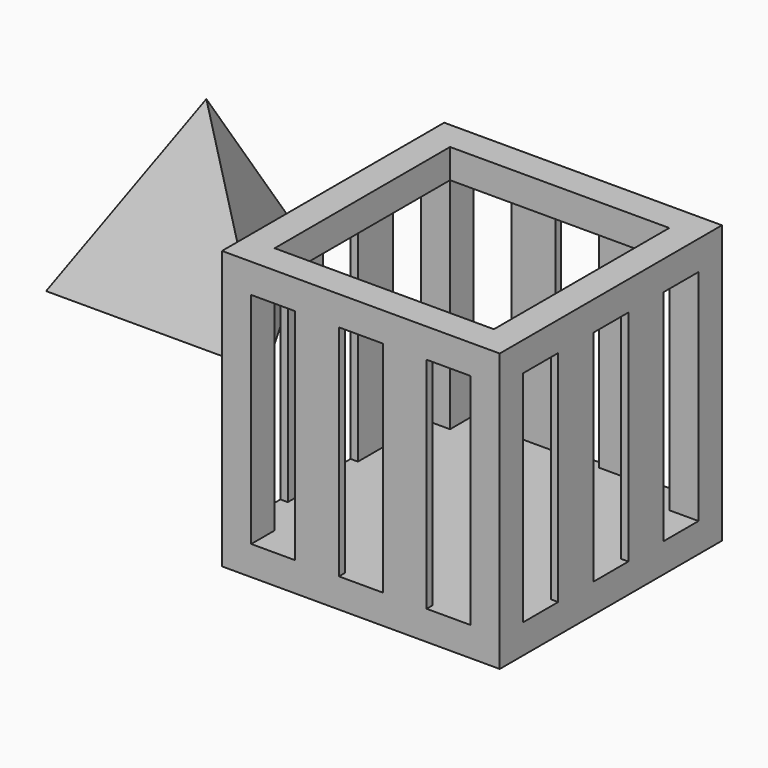
from build123d import *

# Parameters (mm, degrees)
F0_W      = 76
F0_H      = 76
F1_DEPTH  = 76
F2_W      = 60
F2_H      = 60
F3_DEPTH  = 68
F4_W      = 12
F4_H      = 60
F5_DEPTH  = 100
F6_W      = 12
F6_H      = 60
F7_DEPTH  = 6
F8_W      = 12
F8_H      = 60
F9_DEPTH  = 6
F10_W     = 12
F10_H     = 60
F11_DEPTH = 99
F12_W     = 12
F12_H     = 60
F13_DEPTH = 6
F14_W     = 12
F14_H     = 60
F15_DEPTH = 6
F17_DEPTH = 48.9897948557
F20_W     = 96.6173894703
F20_H     = 69.0555498004
F21_DEPTH = 25
F23_W     = 74.8236617073
F23_H     = 72.9810190387
F24_DEPTH = 25
F26_W     = 108.0368701369
F26_H     = 112.1664643288
F27_DEPTH = 25


# Not quite as in the source:
# - a feature names something its author has since deleted; it is built from what else it names


with BuildPart() as f1:
    # F0 (on Right) → F1 (new body)
    with BuildSketch(Plane.YZ):
        with Locations((-38, 38)):
            Rectangle(F0_W, F0_H)
    extrude(amount=F1_DEPTH)

    # F2 (on face) → F3 (cut)
    with BuildSketch(Plane.XY.offset(76)):
        with Locations((38, -38)):
            Rectangle(F2_W, F2_H)
    extrude(amount=-F3_DEPTH, mode=Mode.SUBTRACT)

    # F4 (on face) → F5 (cut)
    with BuildSketch(Plane.XZ.offset(76)):
        with Locations((14, 38)):
            Rectangle(F4_W, F4_H)
        with Locations((38, 38)):
            Rectangle(F4_W, F4_H)
        with Locations((62, 38)):
            Rectangle(F4_W, F4_H)
    extrude(amount=-F5_DEPTH, mode=Mode.SUBTRACT)

    # F6 (on face) → F7 (cut)
    with BuildSketch(Plane(origin=(0, -68, 0), x_dir=(-1, 0, 0), z_dir=(0, 1, 0))):
        with Locations((-50, 38)):
            Rectangle(F6_W, F6_H)
        with Locations((-26, 38)):
            Rectangle(F6_W, F6_H)
    extrude(amount=-F7_DEPTH, mode=Mode.SUBTRACT)

    # F8 (on face) → F9 (cut)
    with BuildSketch(Plane.XZ.offset(8)):
        with Locations((50, 38)):
            Rectangle(F8_W, F8_H)
        with Locations((26, 38)):
            Rectangle(F8_W, F8_H)
    extrude(amount=-F9_DEPTH, mode=Mode.SUBTRACT)

    # F10 (on face) → F11 (cut)
    with BuildSketch(Plane(origin=(0, 0, 0), x_dir=(0, -1, 0), z_dir=(-1, 0, 0))):
        with Locations((14, 38)):
            Rectangle(F10_W, F10_H)
        with Locations((38, 38)):
            Rectangle(F10_W, F10_H)
        with Locations((62, 38)):
            Rectangle(F10_W, F10_H)
    extrude(amount=-F11_DEPTH, mode=Mode.SUBTRACT)

    # F12 (on face) → F13 (cut)
    with BuildSketch(Plane.YZ.offset(8)):
        with Locations((-26, 38)):
            Rectangle(F12_W, F12_H)
        with Locations((-50, 38)):
            Rectangle(F12_W, F12_H)
    extrude(amount=-F13_DEPTH, mode=Mode.SUBTRACT)

    # F14 (on face) → F15 (cut)
    with BuildSketch(Plane(origin=(68, 0, 0), x_dir=(0, -1, 0), z_dir=(-1, 0, 0))):
        with Locations((50, 38)):
            Rectangle(F14_W, F14_H)
        with Locations((26, 38)):
            Rectangle(F14_W, F14_H)
    extrude(amount=-F15_DEPTH, mode=Mode.SUBTRACT)


with BuildPart() as f17:
    # F16 (on Top) → F17 (new body)
    with BuildSketch(Plane.XY):
        Polygon((-63.9376926764, 25.9807621135), (-78.9376926764, 17.3205080757), (-48.9376926764, 0), align=None)
        Polygon((-78.9376926764, 51.9615242271), (-78.9376926764, 17.3205080757), (-63.9376926764, 25.9807621135), align=None)
        Polygon((-78.9376926764, 51.9615242271), (-93.9376926764, 25.9807621135), (-78.9376926764, 17.3205080757), align=None)
        Polygon((-93.9376926764, 25.9807621135), (-108.9376926764, 0), (-78.9376926764, 17.3205080757), align=None)
        Polygon((-78.9376926764, 17.3205080757), (-108.9376926764, 0), (-78.9376926764, 0), align=None)
        Polygon((-78.9376926764, 17.3205080757), (-78.9376926764, 0), (-48.9376926764, 0), align=None)
    extrude(amount=F17_DEPTH)

    # F20 (on 3pt) → F21 (cut)
    with BuildSketch(Plane(origin=(-72.6251284509, 41.9301374611, 29.6490845348), x_dir=(0.4364357805, 0.8819171037, -0.1781741613), z_dir=(0.8164965809, -0.4714045208, -0.3333333333))):
        with Locations((-29.2243789881, -11.6772539914)):
            Rectangle(F20_W, F20_H)
    extrude(amount=-F21_DEPTH, mode=Mode.SUBTRACT)

    # F23 (on 3pt) → F24 (cut)
    with BuildSketch(Plane(origin=(-32.6251284509, -18.8361266935, -13.3191529162), x_dir=(-0.4364357805, 0.8819171037, -0.1781741613), z_dir=(0.8164965809, 0.4714045208, 0.3333333333))):
        with Locations((46.6394056566, 41.2203946617)):
            Rectangle(F23_W, F23_H)
    extrude(amount=F24_DEPTH, mode=Mode.SUBTRACT)

    # F26 (on 3pt) → F27 (cut)
    with BuildSketch(Plane(origin=(0, 0, 0), x_dir=(-1, 0, 0), z_dir=(0, 0.9428090416, -0.3333333333))):
        with Locations((71.1465058848, 24.1519138217)):
            Rectangle(F26_W, F26_H)
    extrude(amount=-F27_DEPTH, mode=Mode.SUBTRACT)


solid = Compound([f1.part, f17.part])
